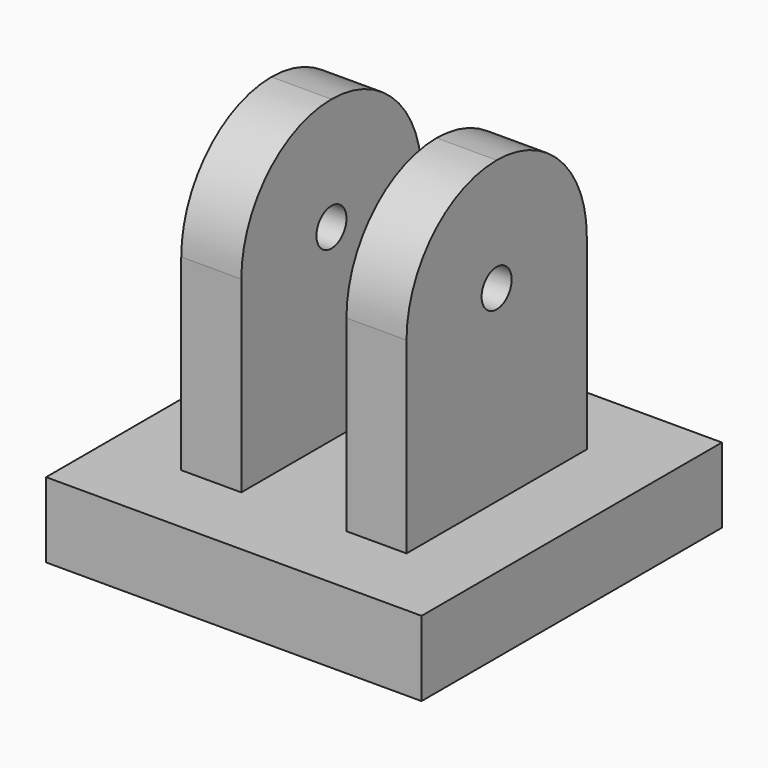
from build123d import *

# Parameters (mm, degrees)
F0_W     = 50
F0_H     = 50
F1_DEPTH = 10
F2_W     = 8
F2_H     = 30
F3_DEPTH = 40
F4_R     = 14.99999
F6_D     = 5


# Not quite as in the source:
# - a fillet or chamfer is up to 0.001 mm smaller than in the source, because OpenCascade refuses the exact size


with BuildPart() as f1:
    # F0 (on Top) → F1 (new body)
    with BuildSketch(Plane.XY):
        with Locations((0.8760243654, 3.7264487195)):
            Rectangle(F0_W, F0_H)
    extrude(amount=F1_DEPTH)

    # F2 (on face) → F3 (join)
    with BuildSketch(Plane.XY.offset(10)):
        with Locations((11.8760243654, 3.7264487195)):
            Rectangle(F2_W, F2_H)
        with Locations((-10.1239756346, 3.7264487195)):
            Rectangle(F2_W, F2_H)
    extrude(amount=F3_DEPTH)

    # F4 (radius 15 in the source; OpenCascade refuses exactly that, so slightly less here)
    f4_edges = [f1.edges().sort_by_distance(p)[0] for p in [
        (-10.123976, -11.273551, 50),
        (11.876024, -11.273551, 50),
        (11.876024, 18.726449, 50),
        (-10.123976, 18.726449, 50),
    ]]
    fillet(f4_edges, radius=F4_R)

    # F6 (through all)
    with Locations(Plane.YZ.offset(15.8760243654)):
        with Locations((3.7264487195, 35)):
            Hole(F6_D / 2)


solid = f1.part
